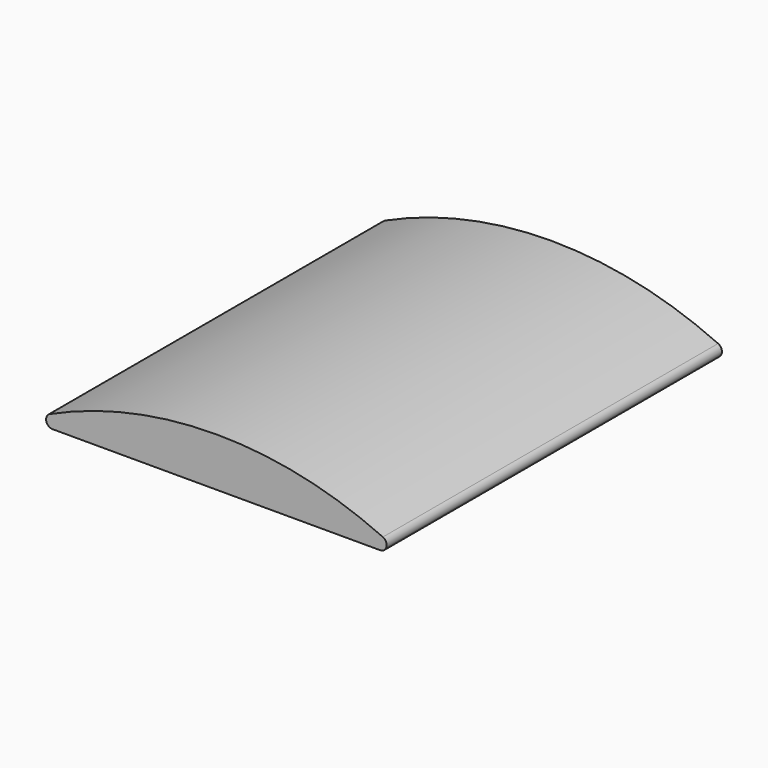
from build123d import *

# Parameters (mm, degrees)
F1_DEPTH = 101.6
F2_F1_R  = 1.5875
F2_F2_R  = 1.5875


with BuildPart() as f1:
    # F0 (on Front) → F1 (new body)
    with BuildSketch(Plane.XZ):
        with BuildLine():
            ThreePointArc((47.5763678551, 0), (1.1439528316, 11.8225265642), (-45.2884621918, 0))
            Line((-45.2884621918, 0), (47.5763678551, 0))
        make_face()
    extrude(amount=-F1_DEPTH)

    # F2: fillet of radius 1.5875 on 2 edges, made by hand

    # F2_f1
    f2_f1_edges = [f1.edges().sort_by_distance(p)[0] for p in [
        (-45.2884621918, 50.8, 0),
    ]]
    fillet(f2_f1_edges, radius=F2_F1_R)

    # F2_f2
    f2_f2_edges = [f1.edges().sort_by_distance(p)[0] for p in [
        (47.5763678551, 50.8, 0),
    ]]
    fillet(f2_f2_edges, radius=F2_F2_R)


solid = f1.part
